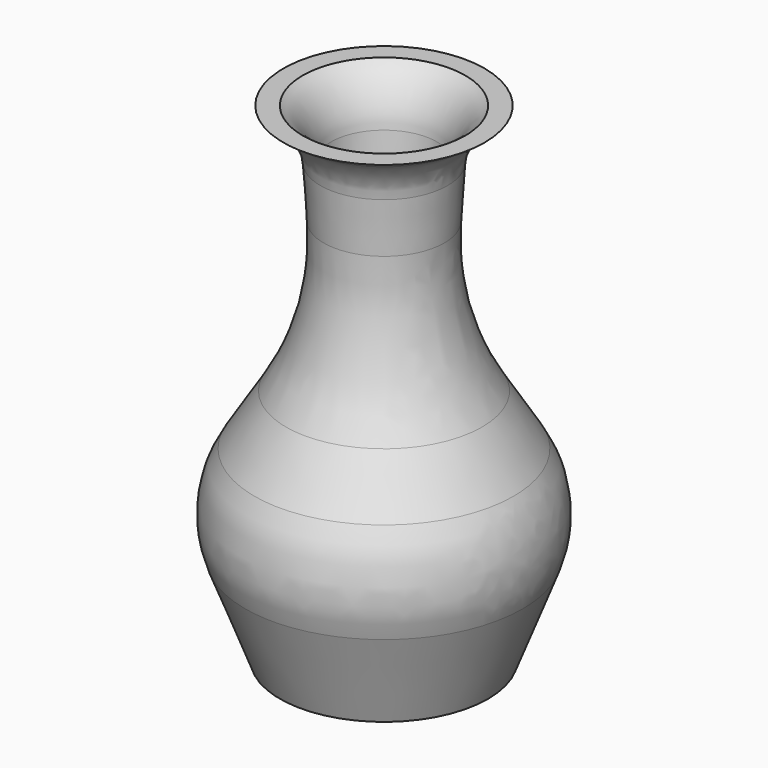
from build123d import *

# Parameters (mm, degrees)
F2_R = 13.0661787558
F3_R = 30.5326661472
F4_R = 6.4496868792
F5_T = 1.27


# Not quite as in the source:
# - a shell that OpenCascade refuses in one call is made with other operations: the cavity is built on its own and cut out


with BuildPart() as f1:
    # F0 (on Front) → F1 (revolve)
    with BuildSketch(Plane.XZ):
        Polygon((0, 58.8393360376), (0, 0), (12.5450463966, 0), (19.0413612872, 16.967702657), (6.6549694166, 36.8729744223), (7.8558586538, 56.0485236347), (12.1103581041, 58.8393360376), align=None)
    revolve(axis=Axis((0, 0, 29.4196680188), (0, 0, -1)))

    # F2
    f2_edges = [f1.edges().sort_by_distance(p)[0] for p in [
        (-19.041361, 0, 16.967703),
    ]]
    fillet(f2_edges, radius=F2_R)

    # F3
    f3_edges = [f1.edges().sort_by_distance(p)[0] for p in [
        (-6.654969, 0, 36.872974),
    ]]
    fillet(f3_edges, radius=F3_R)

    # F4
    f4_edges = [f1.edges().sort_by_distance(p)[0] for p in [
        (-7.855859, 0, 56.048524),
    ]]
    fillet(f4_edges, radius=F4_R)

    # F5: shell of thickness 1.27, made by hand


with BuildPart() as f5_core1:
    # F5_t2: copy of F1
    add(f1.part)

    # the walls: a layer under each face that stays
    f5_faces = [f5_core1.faces().sort_by_distance(p)[0] for p in [
        (-7.4598050795, 0, 49.724422652),
        (-8.5147014286, 0, 55.6656825004),
        (-8.1326981188, 0, 37.2456508864),
        (-11.3320158511, 0, 58.3287689924),
        (-13.7131490398, 0, 25.5302860078),
        (-17.5243000505, 0, 16.8223934121),
        (-14.6325546639, 0, 5.4523557079),
        (0, 0, 0),
    ]]
    thicken(f5_faces, amount=-F5_T, mode=Mode.SUBTRACT)


with BuildPart() as f1_1:
    add(f1.part)

    # what is left inside the walls is the cavity
    f5_cavity = [f5_core1.part.solids().sort_by_distance(p)[0] for p in [
        (-8.12206, -14.071681, 16.700091),
    ]]
    add(f5_cavity, mode=Mode.SUBTRACT)


solid = f1_1.part
